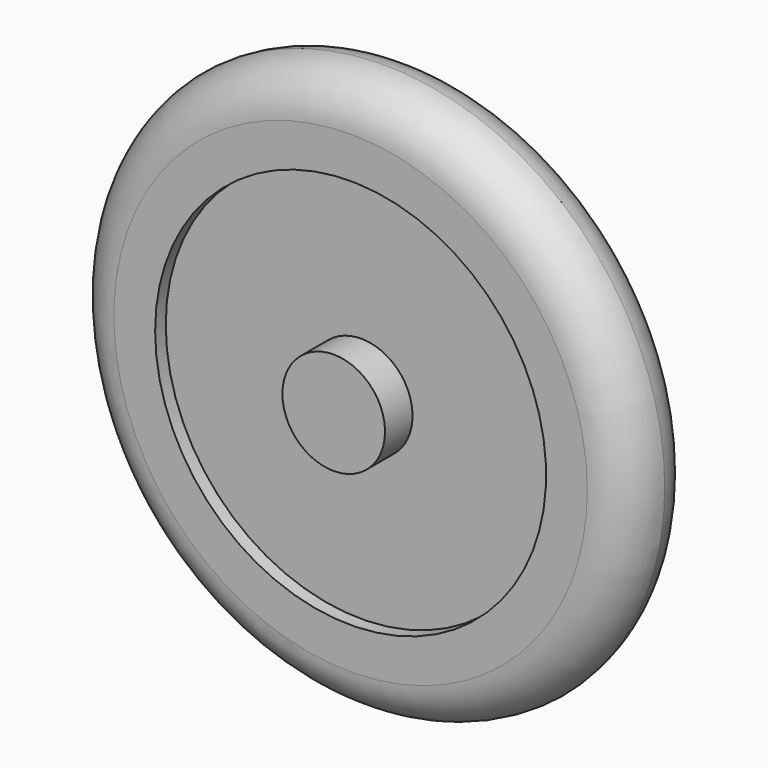
from build123d import *

# Parameters (mm, degrees)
F0_R     = 158.75
F1_DEPTH = 23.495
F3_R     = 110.49
F3_R_2   = 29
F4_DEPTH = 7.5
F5_DEPTH = 11.945


# Not quite as in the source:
# - a fillet or chamfer that OpenCascade refuses, or shapes differently, is made with other operations: its cross-section is extruded or revolved along the edge and cut away or added


with BuildPart() as f1:
    # F0 (on Front) → F1 (new body)
    with BuildSketch(Plane.XZ):
        Circle(F0_R)
    extrude(amount=F1_DEPTH)

    # F2: fillet of radius 25 on 1 edges, made by hand

    # F2_s1 → F2_t2 (revolve, cut)
    with BuildSketch(Plane.XY):
        with BuildLine():
            ThreePointArc((158.75, -23.495), (150.9326547089, -6.7980083507), (133.7953416172, 0))
            Line((133.7953416172, 0), (158.75, 0))
            Line((158.75, 0), (158.75, -23.495))
        make_face()
    revolve(axis=Axis((0, 0, 0), (0, -1, 0)), mode=Mode.SUBTRACT)

    # F3 (on face) → F4 (cut)
    with BuildSketch(Plane(origin=(0, 0, 0), x_dir=(-1, 0, 0), z_dir=(0, 1, 0))):
        Circle(F3_R)
        Circle(F3_R_2, mode=Mode.SUBTRACT)
    extrude(amount=-F4_DEPTH, mode=Mode.SUBTRACT)

    # F5 (add): a face of the model
    f5_faces = [f1.faces().sort_by_distance(p)[0] for p in [
        (0, 0, 0),
    ]]
    extrude(f5_faces, amount=F5_DEPTH)

    # F6: F1 across face


with BuildPart() as f1_1:
    add(f1.part)
    add(f1.part.mirror(Plane.XZ.offset(23.495)))


solid = f1_1.part
